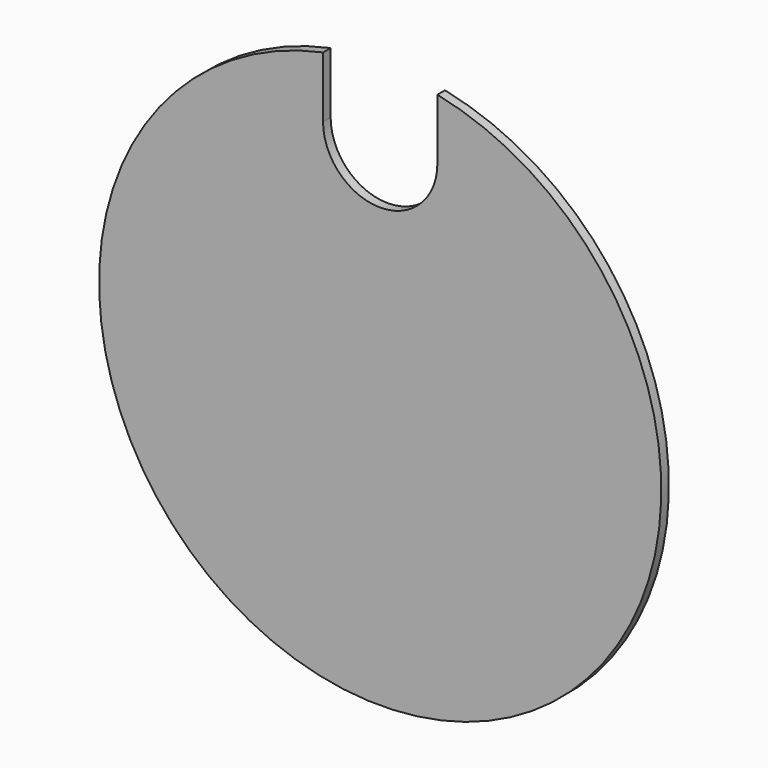
from build123d import *

# Parameters (mm, degrees)
F1_DEPTH = 1


# Not quite as in the source:
# - ends of sketch curves that miss each other by under 0.0002 mm in the source are joined


with BuildPart() as f1:
    # F0 (on Front) → F1 (new body)
    with BuildSketch(Plane.XZ):
        with BuildLine():
            ThreePointArc((-5.9999924445, 28.8833877976), (-18.6178707548, -22.8828514079), (29.5, 0))
            ThreePointArc((29.5, 0), (22.8828562781, 18.617864769), (6.0000075555, 28.8833846586))
            Line((6.0000075555, 28.8833846586), (6.0000075555, 22.5))
            ThreePointArc((6.0000075555, 22.5), (5.9999981111, 22.4952390788), (5.9999924445, 22.4904781605))
            ThreePointArc((5.9999924445, 22.4904781605), (1.2e-08, 16.5), (-5.9999924445, 22.4904781366))
            Line((-5.9999924445, 22.4904781366), (-5.9999924445, 28.8833877976))
        make_face()
    extrude(amount=F1_DEPTH)


solid = f1.part
